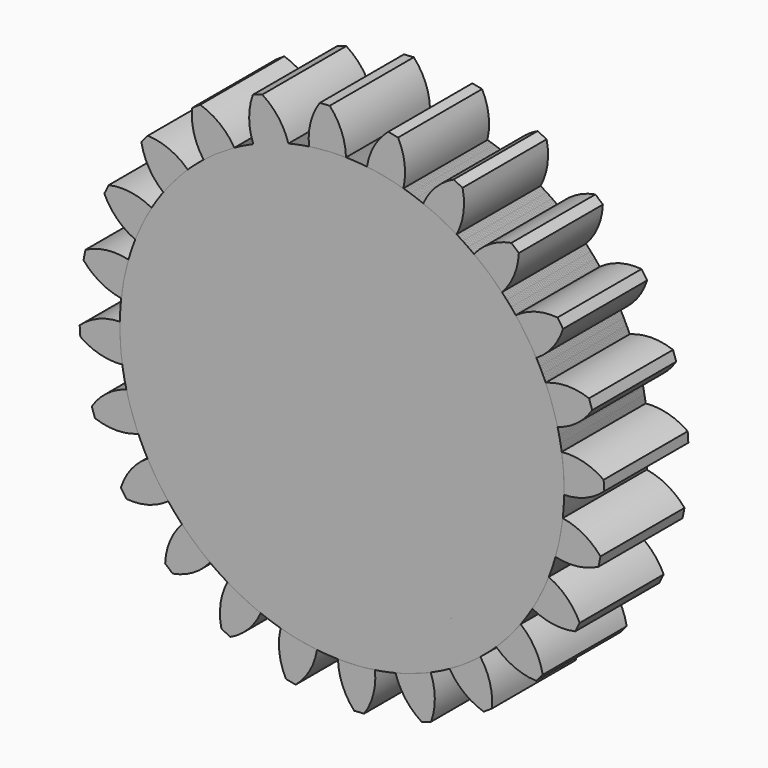
from build123d import *

# Parameters (mm, degrees)
F1_DEPTH = 25.4
F2_COUNT = 24
F2_ANGLE = 345


with BuildPart() as f1:
    # F0 (on Front) → F1 (new body)
    with BuildSketch(Plane.XZ):
        with BuildLine():
            ThreePointArc((-7.9754928515, 53.1256750995), (-3.5135215054, 53.6059792153), (0.9729693247, 53.7121882974))
            ThreePointArc((0.9729693247, 53.7121882974), (-0.1110694251, 58.9274956992), (-2.955610766, 63.4311781776))
            Line((-2.955610766, 63.4311781776), (-5.3491050493, 63.2743002741))
            ThreePointArc((-5.3491050493, 63.2743002741), (-7.5814624199, 58.4378602737), (-7.9754928515, 53.1256750995))
        make_face()
        with BuildLine():
            ThreePointArc((-7.9754928515, 53.1256750995), (-35.053490479, -40.7087047969), (53.721, 0))
            ThreePointArc((53.721, 0), (38.3289363673, 37.6409149457), (0.9729693247, 53.7121882974))
            ThreePointArc((0.9729693247, 53.7121882974), (-3.5135215054, 53.6059792153), (-7.9754928515, 53.1256750995))
        make_face()
    extrude(amount=F1_DEPTH)


with BuildPart() as f2_1:
    # F2: instance of F1
    add(f1.part.rotate(Axis((0, 0, 0), (0, 1, 0)), 1 * F2_ANGLE / (F2_COUNT - 1)))


with BuildPart() as f2_2:
    # F2: instance of F1
    add(f1.part.rotate(Axis((0, 0, 0), (0, 1, 0)), 2 * F2_ANGLE / (F2_COUNT - 1)))


with BuildPart() as f2_3:
    # F2: instance of F1
    add(f1.part.rotate(Axis((0, 0, 0), (0, 1, 0)), 3 * F2_ANGLE / (F2_COUNT - 1)))


with BuildPart() as f2_4:
    # F2: instance of F1
    add(f1.part.rotate(Axis((0, 0, 0), (0, 1, 0)), 4 * F2_ANGLE / (F2_COUNT - 1)))


with BuildPart() as f2_5:
    # F2: instance of F1
    add(f1.part.rotate(Axis((0, 0, 0), (0, 1, 0)), 5 * F2_ANGLE / (F2_COUNT - 1)))


with BuildPart() as f2_6:
    # F2: instance of F1
    add(f1.part.rotate(Axis((0, 0, 0), (0, 1, 0)), 6 * F2_ANGLE / (F2_COUNT - 1)))


with BuildPart() as f2_7:
    # F2: instance of F1
    add(f1.part.rotate(Axis((0, 0, 0), (0, 1, 0)), 7 * F2_ANGLE / (F2_COUNT - 1)))


with BuildPart() as f2_8:
    # F2: instance of F1
    add(f1.part.rotate(Axis((0, 0, 0), (0, 1, 0)), 8 * F2_ANGLE / (F2_COUNT - 1)))


with BuildPart() as f2_9:
    # F2: instance of F1
    add(f1.part.rotate(Axis((0, 0, 0), (0, 1, 0)), 9 * F2_ANGLE / (F2_COUNT - 1)))


with BuildPart() as f2_10:
    # F2: instance of F1
    add(f1.part.rotate(Axis((0, 0, 0), (0, 1, 0)), 10 * F2_ANGLE / (F2_COUNT - 1)))


with BuildPart() as f2_11:
    # F2: instance of F1
    add(f1.part.rotate(Axis((0, 0, 0), (0, 1, 0)), 11 * F2_ANGLE / (F2_COUNT - 1)))


with BuildPart() as f2_12:
    # F2: instance of F1
    add(f1.part.rotate(Axis((0, 0, 0), (0, 1, 0)), 12 * F2_ANGLE / (F2_COUNT - 1)))


with BuildPart() as f2_13:
    # F2: instance of F1
    add(f1.part.rotate(Axis((0, 0, 0), (0, 1, 0)), 13 * F2_ANGLE / (F2_COUNT - 1)))


with BuildPart() as f2_14:
    # F2: instance of F1
    add(f1.part.rotate(Axis((0, 0, 0), (0, 1, 0)), 14 * F2_ANGLE / (F2_COUNT - 1)))


with BuildPart() as f2_15:
    # F2: instance of F1
    add(f1.part.rotate(Axis((0, 0, 0), (0, 1, 0)), 15 * F2_ANGLE / (F2_COUNT - 1)))


with BuildPart() as f2_16:
    # F2: instance of F1
    add(f1.part.rotate(Axis((0, 0, 0), (0, 1, 0)), 16 * F2_ANGLE / (F2_COUNT - 1)))


with BuildPart() as f2_17:
    # F2: instance of F1
    add(f1.part.rotate(Axis((0, 0, 0), (0, 1, 0)), 17 * F2_ANGLE / (F2_COUNT - 1)))


with BuildPart() as f2_18:
    # F2: instance of F1
    add(f1.part.rotate(Axis((0, 0, 0), (0, 1, 0)), 18 * F2_ANGLE / (F2_COUNT - 1)))


with BuildPart() as f2_19:
    # F2: instance of F1
    add(f1.part.rotate(Axis((0, 0, 0), (0, 1, 0)), 19 * F2_ANGLE / (F2_COUNT - 1)))


with BuildPart() as f2_20:
    # F2: instance of F1
    add(f1.part.rotate(Axis((0, 0, 0), (0, 1, 0)), 20 * F2_ANGLE / (F2_COUNT - 1)))


with BuildPart() as f2_21:
    # F2: instance of F1
    add(f1.part.rotate(Axis((0, 0, 0), (0, 1, 0)), 21 * F2_ANGLE / (F2_COUNT - 1)))


with BuildPart() as f2_22:
    # F2: instance of F1
    add(f1.part.rotate(Axis((0, 0, 0), (0, 1, 0)), 22 * F2_ANGLE / (F2_COUNT - 1)))


with BuildPart() as f2_23:
    # F2: instance of F1
    add(f1.part.rotate(Axis((0, 0, 0), (0, 1, 0)), 23 * F2_ANGLE / (F2_COUNT - 1)))


solid = Compound([f1.part, f2_1.part, f2_2.part, f2_3.part, f2_4.part, f2_5.part, f2_6.part, f2_7.part, f2_8.part, f2_9.part, f2_10.part, f2_11.part, f2_12.part, f2_13.part, f2_14.part, f2_15.part, f2_16.part, f2_17.part, f2_18.part, f2_19.part, f2_20.part, f2_21.part, f2_22.part, f2_23.part])
